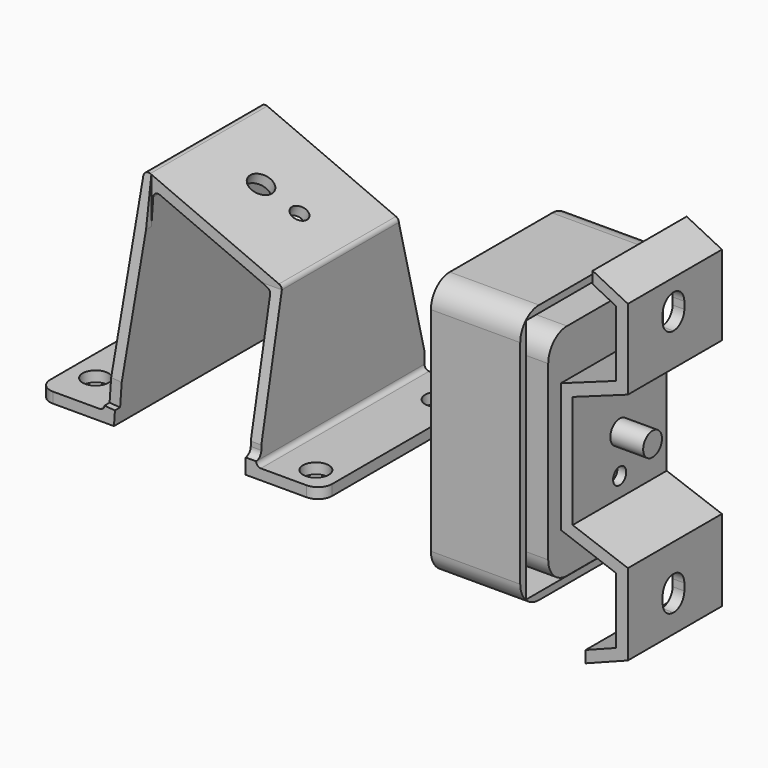
from build123d import *

# Parameters (mm, degrees)
F0_W        = 27.5
F0_H        = 4.5
F1_DEPTH    = 89.5
F2_R        = 2
F4_DEPTH    = 55.5
F5_T1_DEPTH = 4.5
F7_DEPTH    = 25
F8_R        = 5.5
F9_DEPTH    = 5
F10_R       = 5.5
F11_DEPTH   = 5
F12_R       = 5
F12_R_2     = 3.5
F13_DEPTH   = 5
F14_R       = 6
F16_DEPTH   = 61
F17_R       = 5
F18_DEPTH   = 20
F17_R_2     = 3.5
F19_DEPTH   = 2.25
F20_R       = 5
F21_DEPTH   = 26
F20_R_2     = 3.5
F22_DEPTH   = 5.5
F23_R       = 10
F25_W       = 74.5
F25_H       = 110.5
F25_R       = 5
F25_R_2     = 3.5
F26_DEPTH   = 38
F27_W       = 68.5
F27_H       = 104.5
F27_R       = 5
F27_R_2     = 3.5
F28_DEPTH   = 35
F29_R       = 10
F31_W       = 50
F31_H       = 148
F31_R       = 3.5
F31_R_2     = 5
F32_DEPTH   = 28.5
F34_DEPTH   = 50
F36_DEPTH   = 5


# Not quite as in the source:
# - a fillet or chamfer that OpenCascade refuses, or shapes differently, is made with other operations: its cross-section is extruded or revolved along the edge and cut away or added


with BuildPart() as f1:
    # F0 (on Front) → F1 (new body)
    with BuildSketch(Plane.XZ):
        Polygon((-32, 0), (-27.5, 0), (-27.5, 4.5), (-27.5, 66.4633900416), (-86.0427199911, 91.6367596378), (-92.1935500832, 4.5), (-92.4888345559, 0.3168033031), (-92.5, 0), (-88, 0), (-82, 85), (-32, 63.5), align=None)
        with Locations((-13.75, 2.25)):
            Rectangle(F0_W, F0_H)
        Polygon((-120, 0), (-92.5, 0), (-92.4888345559, 0.3168033031), (-92.1935500832, 4.5), (-120, 4.5), align=None)
    extrude(amount=-F1_DEPTH)

    # F2
    f2_edges = [f1.edges().sort_by_distance(p)[0] for p in [
        (-86.04272, 44.75, 91.63676),
        (-82, 44.75, 85),
        (-32, 44.75, 63.5),
        (-27.5, 44.75, 66.46339),
        (-92.19355, 44.75, 4.5),
        (-27.5, 44.75, 4.5),
    ]]
    fillet(f2_edges, radius=F2_R)

    # F3 (on face) → F4 (cut)
    with BuildSketch(Plane.YZ.offset(-27.5)):
        Polygon((89.5, 66.9836661761), (89.5, 90.5244270628), (75.85, 90.5244270628), (75.85, 65.1463278009), (89.5, 65.1463278009), align=None)
        Polygon((89.5, 65.1463278009), (75.85, 65.1463278009), (89.5, 11.5), align=None)
        Polygon((2.75, 11.5), (13.65, 65.1463278009), (0, 65.1463278009), (0, 6.5), (2.75, 6.5), align=None)
        Polygon((13.65, 65.1463278009), (13.65, 90.5244270628), (0, 90.5244270628), (0, 66.9836661761), (0, 65.1463278009), align=None)
    extrude(amount=-F4_DEPTH, mode=Mode.SUBTRACT)

    # F5: fillet of radius 3 on 1 edges, made by hand

    # F5_s2 → F5_t1 (join)
    with BuildSketch(Plane.YZ.offset(-32)):
        with BuildLine():
            ThreePointArc((2.75, 9.4895651858), (1.9579402166, 7.4585555846), (0, 6.5))
            Line((0, 6.5), (2.75, 6.5))
            Line((2.75, 6.5), (2.75, 9.4895651858))
        make_face()
    extrude(amount=F5_T1_DEPTH)

    # F6 (on face) → F7 (cut)
    with BuildSketch(Plane(origin=(-92.0525271107, 0, 6.4978254431), x_dir=(0, -1, 0), z_dir=(-0.9975179223, 0, 0.0704130298))):
        Polygon((-89.5, 9.5350977863), (-76.1650987076, 82.5349474599), (-89.5, 82.5349474599), align=None)
        Polygon((-89.5, 84.4233556199), (-75.85, 84.4233556199), (-75.85, 87.4233556199), (-89.5, 87.4233556199), (-89.5, 84.5349474599), align=None)
        Polygon((-75.85, 84.2599064816), (-75.85, 84.4233556199), (-89.5, 84.4233556199), (-89.5, 82.5349474599), (-76.1650987076, 82.5349474599), align=None)
        Polygon((-13.65, 87.4233556199), (-13.65, 84.4233556199), (0, 84.4233556199), (0, 84.5349474599), (0, 87.4233556199), align=None)
        Polygon((-13.65, 84.4233556199), (-13.65, 84.2599064816), (-13.398382717, 82.5349474599), (0, 82.5349474599), (0, 84.4233556199), align=None)
        Polygon((0, 82.5349474599), (-13.398382717, 82.5349474599), (-2.75, 9.5350977863), (-2.75, 7.5296530276), (-2.75, -0.1389965028), (0, -0.1389965028), align=None)
    extrude(amount=-F7_DEPTH, mode=Mode.SUBTRACT)

    # F8 (on face) → F9 (cut)
    with BuildSketch(Plane.XY.offset(4.5)):
        with Locations((-10.5, 10.5)):
            Circle(F8_R)
        with Locations((-10.5, 75.5)):
            Circle(F8_R)
    extrude(amount=-F9_DEPTH, mode=Mode.SUBTRACT)

    # F10 (on face) → F11 (cut)
    with BuildSketch(Plane.XY.offset(4.5)):
        with Locations((-109, 16.5)):
            Circle(F10_R)
        with Locations((-109, 78.5)):
            Circle(F10_R)
    extrude(amount=-F11_DEPTH, mode=Mode.SUBTRACT)

    # F12 (on face) → F13 (cut)
    with BuildSketch(Plane(origin=(19.8282620625, 0, 46.1122373547), x_dir=(0.9186691876, 0, -0.3950277507), z_dir=(0.3950277507, 0, 0.9186691876))):
        with Locations((-88.3164328594, 44.85)):
            Circle(F12_R)
        with Locations((-71.8164328594, 46.35)):
            Circle(F12_R_2)
    extrude(amount=-F13_DEPTH, mode=Mode.SUBTRACT)

    # F14
    f14_edges = [f1.edges().sort_by_distance(p)[0] for p in [
        (0, 89.5, 2.25),
        (0, 0, 2.25),
        (-120, 0, 2.25),
        (-120, 89.5, 2.25),
    ]]
    fillet(f14_edges, radius=F14_R)


with BuildPart() as f16:
    # F15 (on Front) → F16 (new body)
    with BuildSketch(Plane.XZ):
        Polygon((53.25, 0), (75, 0), (96.75, 0), (96.75, 93.5), (53.25, 93.5), align=None)
    extrude(amount=-F16_DEPTH)

    # F17 (on face) → F18 (join)
    with BuildSketch(Plane.YZ.offset(96.75)):
        with Locations((30.5, 47.5)):
            Circle(F17_R)
    extrude(amount=F18_DEPTH)

    # F17 (on face) → F19 (join)
    with BuildSketch(Plane.YZ.offset(96.75)):
        with Locations((30.5, 47.5)):
            Circle(F17_R)
        with Locations((30.5, 31)):
            Circle(F17_R_2)
    extrude(amount=F19_DEPTH)

    # F20 (on face) → F21 (join)
    with BuildSketch(Plane(origin=(53.25, 0, 0), x_dir=(0, -1, 0), z_dir=(-1, 0, 0))):
        with Locations((-30.5, 36.5)):
            Circle(F20_R)
    extrude(amount=F21_DEPTH)

    # F20 (on face) → F22 (join)
    with BuildSketch(Plane(origin=(53.25, 0, 0), x_dir=(0, -1, 0), z_dir=(-1, 0, 0))):
        with Locations((-30.5, 36.5)):
            Circle(F20_R)
        with Locations((-30.5, 53)):
            Circle(F20_R_2)
    extrude(amount=F22_DEPTH)

    # F23
    f23_edges = [f16.edges().sort_by_distance(p)[0] for p in [
        (75, 0, 93.5),
        (75, 61, 93.5),
        (75, 61, 0),
        (75, 0, 0),
    ]]
    fillet(f23_edges, radius=F23_R)


with BuildPart() as f26:
    # F25 (on offset) → F26 (new body)
    with BuildSketch(Plane(origin=(52.25, 0, 0), x_dir=(0, -1, 0), z_dir=(-1, 0, 0))):
        with Locations((-30.5, 46.75)):
            Rectangle(F25_W, F25_H)
        with Locations((-30.5, 36.5)):
            Circle(F25_R, mode=Mode.SUBTRACT)
        with Locations((-30.5, 53)):
            Circle(F25_R_2, mode=Mode.SUBTRACT)
    extrude(amount=-F26_DEPTH)

    # F27 (on face) → F28 (cut)
    with BuildSketch(Plane.YZ.offset(90.25)):
        with Locations((30.5, 46.75)):
            Rectangle(F27_W, F27_H)
        with Locations((30.5, 36.5)):
            Circle(F27_R, mode=Mode.SUBTRACT)
        with Locations((30.5, 53)):
            Circle(F27_R_2, mode=Mode.SUBTRACT)
    extrude(amount=-F28_DEPTH, mode=Mode.SUBTRACT)

    # F29
    f29_edges = [f26.edges().sort_by_distance(p)[0] for p in [
        (71.25, -6.75, 102),
        (71.25, 67.75, 102),
        (71.25, 67.75, -8.5),
        (71.25, -6.75, -8.5),
    ]]
    fillet(f29_edges, radius=F29_R)


with BuildPart() as f32:
    # F31 (on offset) → F32 (new body)
    with BuildSketch(Plane.YZ.offset(97.75)):
        with Locations((30.5, 46.75)):
            Rectangle(F31_W, F31_H)
        with Locations((30.5, 31)):
            Circle(F31_R, mode=Mode.SUBTRACT)
        with Locations((30.5, 47.5)):
            Circle(F31_R_2, mode=Mode.SUBTRACT)
    extrude(amount=F32_DEPTH)

    # F33 (on face) → F34 (cut)
    with BuildSketch(Plane.XZ.offset(-5.5)):
        Polygon((111.25, 120.75), (126.25, 113.25), (126.25, 120.75), align=None)
        Polygon((97.75, 120.75), (97.75, 74.25), (121.25, 82.75), (121.25, 110.75), (111.25, 115.75), (111.25, 120.75), align=None)
        Polygon((102.75, 22.7585102126), (126.25, 14.2585102126), (126.25, 79.2414897874), (102.75, 70.7414897874), align=None)
        Polygon((97.75, -27.25), (108.25, -27.25), (108.25, -22.25), (121.25, -17.25), (121.25, 10.75), (97.75, 19.25), align=None)
        Polygon((108.25, -27.25), (126.25, -27.25), (126.25, -20.3269230769), align=None)
    extrude(amount=-F34_DEPTH, mode=Mode.SUBTRACT)

    # F35 (on face) → F36 (cut)
    with BuildSketch(Plane.YZ.offset(126.25)):
        with BuildLine():
            ThreePointArc((29.75, -12.25), (33.8158639918, -10.5658639918), (35.5, -6.5))
            Line((35.5, -6.5), (35.5, -3.5))
            ThreePointArc((35.5, -3.5), (33.8158639918, 0.5658639918), (29.75, 2.25))
            ThreePointArc((29.75, 2.25), (25.6841360082, 0.5658639918), (24, -3.5))
            Line((24, -3.5), (24, -6.5))
            ThreePointArc((24, -6.5), (25.6841360082, -10.5658639918), (29.75, -12.25))
        make_face()
        with BuildLine():
            ThreePointArc((24, 99), (25.6841360082, 94.9341360082), (29.75, 93.25))
            ThreePointArc((29.75, 93.25), (33.8158639918, 94.9341360082), (35.5, 99))
            Line((35.5, 99), (35.5, 102))
            ThreePointArc((35.5, 102), (33.8158639918, 106.0658639918), (29.75, 107.75))
            ThreePointArc((29.75, 107.75), (25.6841360082, 106.0658639918), (24, 102))
            Line((24, 102), (24, 99))
        make_face()
    extrude(amount=-F36_DEPTH, mode=Mode.SUBTRACT)


solid = Compound([f1.part, f16.part, f26.part, f32.part])
